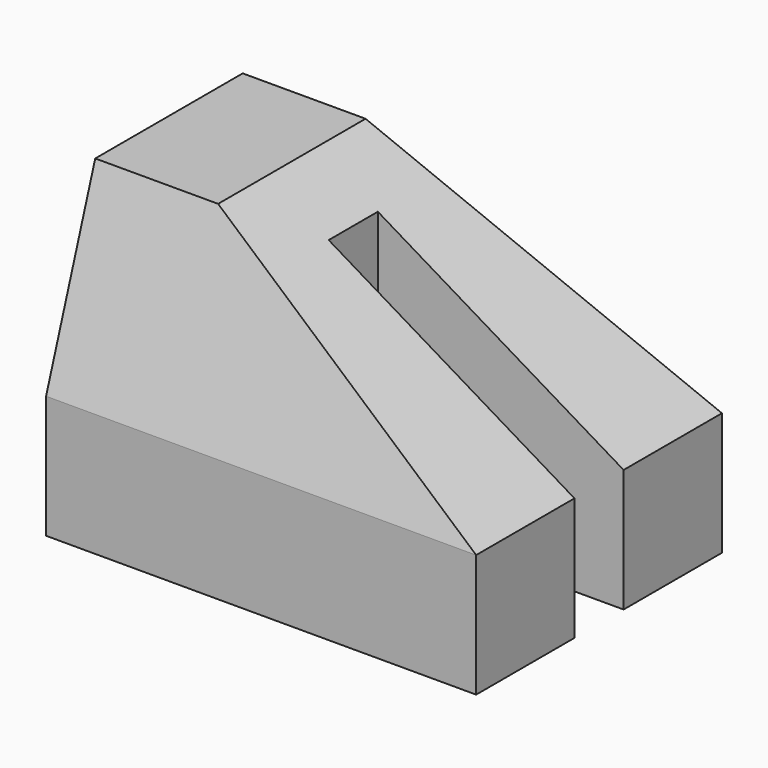
from build123d import *

# Parameters (mm, degrees)
F0_W     = 70
F0_H     = 50
F1_DEPTH = 20
F3_DEPTH = 50
F5_DEPTH = 70.001
F6_W     = 40
F6_H     = 10
F7_DEPTH = 50.001


# Not quite as in the source:
# - a pattern or mirror of a feature is missing from the dataset's text; its kind, count and spacing are read off the source's solid


with BuildPart() as f1:
    # F0 (on Top) → F1 (new body)
    with BuildSketch(Plane.XY):
        with Locations((35, 0)):
            Rectangle(F0_W, F0_H)
    extrude(amount=F1_DEPTH)

    # F2 (on face) → F3 (join, through all)
    with BuildSketch(Plane.XZ.offset(25)):
        Polygon((0, 50), (0, 20), (70, 20), (20, 50), align=None)
    extrude(amount=-F3_DEPTH)

    # F4 (on face) → F5 (cut, through all)
    with BuildSketch(Plane(origin=(0, 0, 0), x_dir=(0, -1, 0), z_dir=(-1, 0, 0))):
        Polygon((25, 20), (25, 50), (15, 50), align=None)
    f5 = extrude(amount=-F5_DEPTH, mode=Mode.SUBTRACT)

    # F5_copies: F5 across plane
    add(f5.mirror(Plane.ZX), mode=Mode.SUBTRACT)

    # F6 (on face) → F7 (cut, through all)
    with BuildSketch(Plane.XY.offset(50)):
        with Locations((50, 0)):
            Rectangle(F6_W, F6_H)
    extrude(amount=-F7_DEPTH, mode=Mode.SUBTRACT)


solid = f1.part
